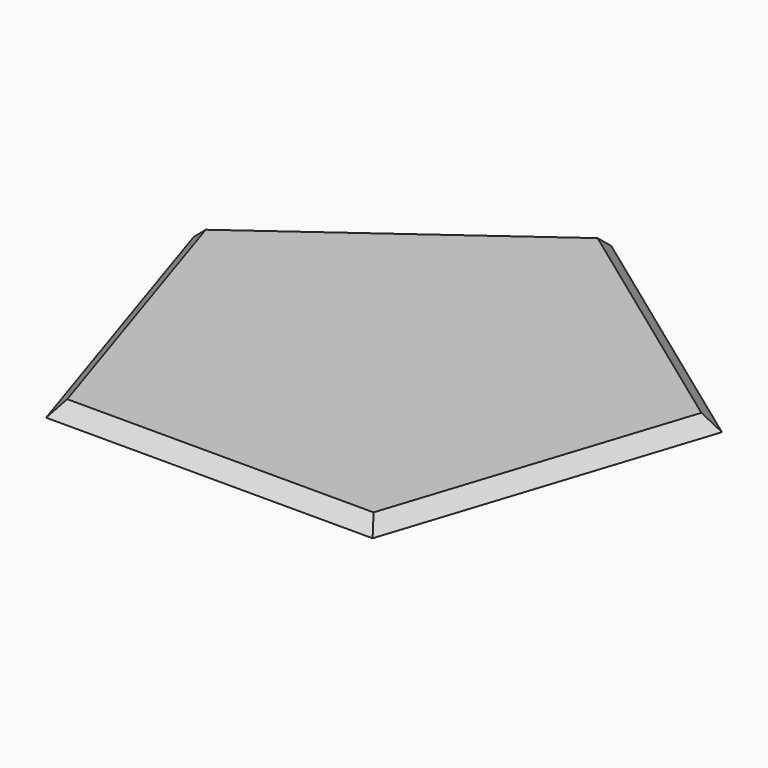
from build123d import *

# Parameters (mm, degrees)
F1_DEPTH = 3.175
F2_SIZE  = 3.17499


# Not quite as in the source:
# - a fillet or chamfer is up to 0.001 mm smaller than in the source, because OpenCascade refuses the exact size


with BuildPart() as f1:
    # F0 (on Top) → F1 (new body)
    with BuildSketch(Plane.XY):
        Polygon((60.3920887847, 19.6225791428), (0, 63.5), (-60.3920887847, 19.6225791428), (-37.3243635206, -51.3725791428), (37.3243635206, -51.3725791428), align=None)
    extrude(amount=F1_DEPTH)

    # F2 (size 3.175 in the source; OpenCascade refuses exactly that, so slightly less here)
    f2_edges = [f1.edges().sort_by_distance(p)[0] for p in [
        (30.196044, 41.56129, 3.175),
        (-30.196044, 41.56129, 3.175),
        (-48.858226, -15.875, 3.175),
        (0, -51.372579, 3.175),
        (48.858226, -15.875, 3.175),
    ]]
    chamfer(f2_edges, length=F2_SIZE)


solid = f1.part
